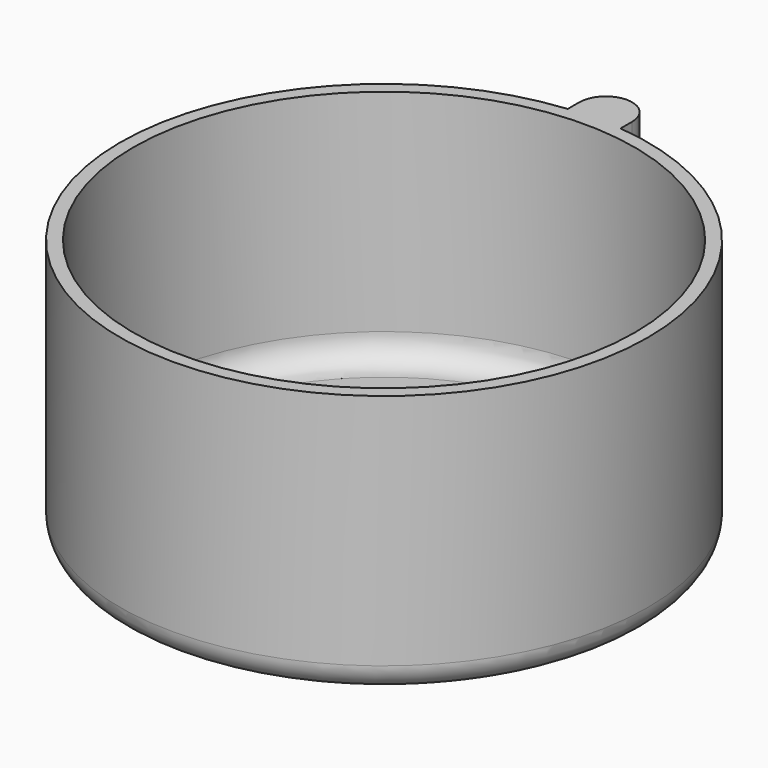
from build123d import *

# Parameters (mm, degrees)
F0_R     = 50.8
F1_DEPTH = 50.8
F2_R     = 48.26
F3_DEPTH = 45.72
F4_R     = 5.08
F5_R     = 5.08
F7_DEPTH = 50.8
F8_R     = 1.27


# Not quite as in the source:
# - the program builds the solid bodies; features that only make, move or delete a surface that nothing else refers to are left out


with BuildPart() as f1:
    # F0 (on Top) → F1 (new body)
    with BuildSketch(Plane.XY):
        Circle(F0_R)
    extrude(amount=F1_DEPTH)

    # F2 (on face) → F3 (cut)
    with BuildSketch(Plane.XY.offset(50.8)):
        Circle(F2_R)
    extrude(amount=-F3_DEPTH, mode=Mode.SUBTRACT)

    # F4
    f4_edges = [f1.edges().sort_by_distance(p)[0] for p in [
        (-48.26, 0, 5.08),
    ]]
    fillet(f4_edges, radius=F4_R)

    # F5
    f5_edges = [f1.edges().sort_by_distance(p)[0] for p in [
        (-50.8, 0, 0),
    ]]
    fillet(f5_edges, radius=F5_R)

    # F6 (on face) → F7 (join)
    with BuildSketch(Plane.XY.offset(50.8)):
        with BuildLine():
            ThreePointArc((5.08, 53.34), (0, 58.42), (-5.08, 53.34))
            Line((-5.08, 53.34), (-5.0849799889, 50.5448610495))
            ThreePointArc((-5.0849799889, 50.5448610495), (-0.002502551, 50.7999999384), (5.08, 50.545361805))
            Line((5.08, 50.545361805), (5.08, 50.8))
            Line((5.08, 50.8), (5.08, 53.34))
        make_face()
    extrude(amount=-F7_DEPTH)

    # F8
    f8_edges = [f1.edges().sort_by_distance(p)[0] for p in [
        (-0.002503, 50.8, 0),
    ]]
    fillet(f8_edges, radius=F8_R)


solid = f1.part
